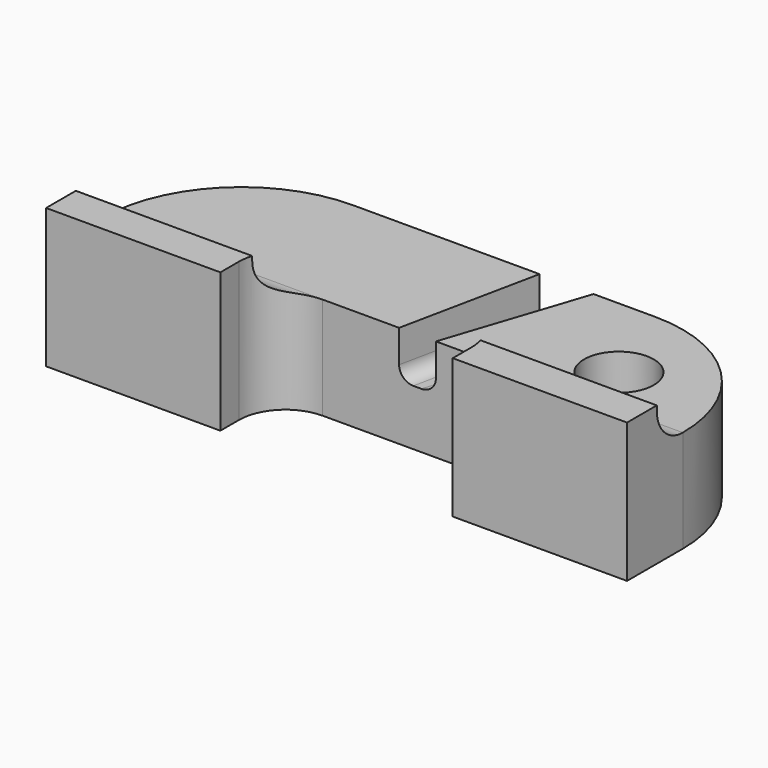
from build123d import *

# Parameters (mm, degrees)
F1_DEPTH = 7.62
F3_DEPTH = 4.572
F4_R     = 0.762
F5_R     = 1.905
F6_DEPTH = 7.621
F8_DEPTH = 31.751


with BuildPart() as f1:
    # F0 (on Top) → F1 (new body)
    with BuildSketch(Plane.XY):
        with BuildLine():
            ThreePointArc((-6.35, 2.54), (-5.6060512242, 4.3360512242), (-3.81, 5.08))
            Line((-3.81, 5.08), (3.81, 5.08))
            ThreePointArc((3.81, 5.08), (5.6060512242, 4.3360512242), (6.35, 2.54))
            Line((6.35, 2.54), (6.35, 1.27))
            Line((6.35, 1.27), (15.875, 1.27))
            Line((15.875, 1.27), (15.875, 5.08))
            ThreePointArc((15.875, 5.08), (13.6431536726, 10.4681536726), (8.255, 12.7))
            Line((8.255, 12.7), (-8.255, 12.7))
            ThreePointArc((-8.255, 12.7), (-13.6431536726, 10.4681536726), (-15.875, 5.08))
            Line((-15.875, 5.08), (-15.875, 1.27))
            Line((-15.875, 1.27), (-6.35, 1.27))
            Line((-6.35, 1.27), (-6.35, 2.54))
        make_face()
    extrude(amount=F1_DEPTH)

    # F2 (on face) → F3 (cut)
    with BuildSketch(Plane.XY.offset(7.62)):
        Polygon((2.153245525, 13.6789603775), (0.3542888121, 5.0024012453), (2.1943775111, 4.5093509644), (4.9747148636, 12.9229499468), align=None)
    extrude(amount=-F3_DEPTH, mode=Mode.SUBTRACT)

    # F4
    f4_edges = [f1.edges().sort_by_distance(p)[0] for p in [
        (1.160325, 8.89, 3.048),
        (3.641996, 8.89, 3.048),
    ]]
    fillet(f4_edges, radius=F4_R)

    # F5 (on face) → F6 (cut, through all)
    with BuildSketch(Plane.XY.offset(7.62)):
        with Locations((10.2573568001, 7.736901287)):
            Circle(F5_R)
    extrude(amount=-F6_DEPTH, mode=Mode.SUBTRACT)

    # F7 (on face) → F8 (cut, through all)
    with BuildSketch(Plane(origin=(-15.875, 0, 0), x_dir=(0, -1, 0), z_dir=(-1, 0, 0))):
        with BuildLine():
            Line((-3.302, 7.62), (-12.7, 7.62))
            Line((-12.7, 7.62), (-12.7, 5.588))
            Line((-12.7, 5.588), (-5.08, 5.588))
            ThreePointArc((-5.08, 5.588), (-3.8227641431, 6.1087641431), (-3.302, 7.366))
            Line((-3.302, 7.366), (-3.302, 7.62))
        make_face()
    extrude(amount=-F8_DEPTH, mode=Mode.SUBTRACT)


solid = f1.part
